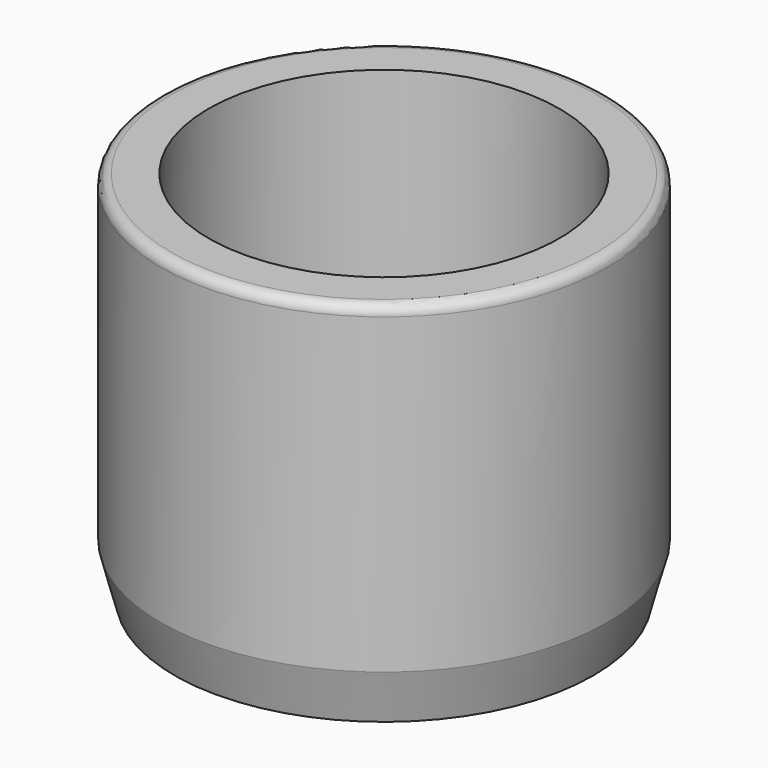
from build123d import *

# Parameters (mm, degrees)
F2_R     = 1.5
F3_DEPTH = 80
F4_R     = 0.5
F5_R     = 1.5
F6_DEPTH = 6.75


# Not quite as in the source:
# - a feature names something its author has since deleted; it is built from what else it names


with BuildPart() as f1:
    # F0 (on Front) → F1 (revolve)
    with BuildSketch(Plane.XZ):
        with BuildLine():
            Line((-8.65, 66), (-11, 66))
            Line((-11, 66), (-11, 50.0923395157))
            Line((-11, 50.0923395157), (-10.3264193874, 47.5785024464))
            Line((-10.3264193874, 47.5785024464), (-2, 47.5785024464))
            Line((-2, 47.5785024464), (-2, 50.8554930795))
            Line((-2, 50.8554930795), (-3, 53))
            Line((-3, 53), (-7.65, 53))
            ThreePointArc((-7.65, 53), (-8.3571067812, 53.2928932188), (-8.65, 54))
            Line((-8.65, 54), (-8.65, 66))
        make_face()
    revolve(axis=Axis((0, 0, 14.8610904367), (0, 0, -1)))

    # F2 (on Top) → F3 (cut)
    with BuildSketch(Plane.XY):
        with Locations((-6.5, 0)):
            Circle(F2_R)
        with BuildLine():
            ThreePointArc((8, 0), (6.5, 1.5), (5, 0))
            ThreePointArc((5, 0), (6.5, -1.5), (8, 0))
        make_face()
    extrude(amount=F3_DEPTH, mode=Mode.SUBTRACT)

    # F4
    f4_edges = [f1.edges().sort_by_distance(p)[0] for p in [
        (11, 0, 66),
    ]]
    fillet(f4_edges, radius=F4_R)

    # F5 (on Right) → F6 (cut, symmetric)
    with BuildSketch(Plane.YZ):
        with Locations((0, 47.5850664079)):
            Circle(F5_R)
    extrude(amount=F6_DEPTH, both=True, mode=Mode.SUBTRACT)


solid = f1.part
